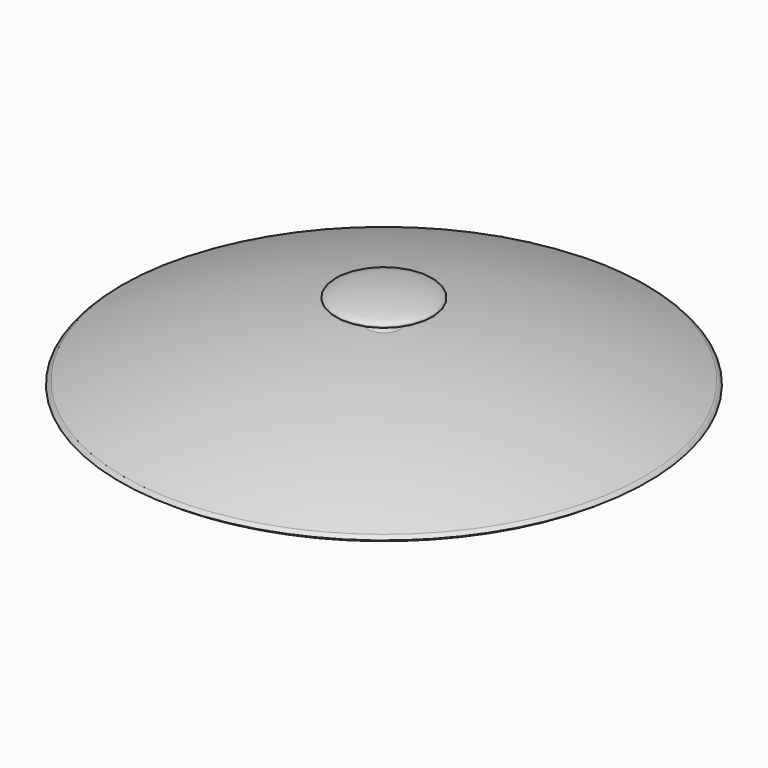
from build123d import *

# Parameters (mm, degrees)
F3_R = 3.175


# Not quite as in the source:
# - a fillet or chamfer that OpenCascade refuses, or shapes differently, is made with other operations: its cross-section is extruded or revolved along the edge and cut away or added


with BuildPart() as f1:
    # F0 (on Front) → F1 (revolve)
    with BuildSketch(Plane.XZ):
        with BuildLine():
            ThreePointArc((-99.06, 0), (-50.3848076923, 13.97), (0, 19.05))
            Line((0, 19.05), (0, 20.9474936326))
            ThreePointArc((0, 20.9474936326), (-1.587572816, 20.9257561642), (-3.175, 20.8951800399))
            ThreePointArc((-3.175, 20.8951800399), (-53.7682024502, 15.2345142884), (-102.54869, 0.6681384411))
            Line((-102.54869, 0.6681384411), (-102.54869, 0))
            Line((-102.54869, 0), (-101.6, 0))
            Line((-101.6, 0), (-99.06, 0))
        make_face()
        with BuildLine():
            ThreePointArc((-101.6, 0), (-100.33, -1.27), (-99.06, 0))
            Line((-99.06, 0), (-101.6, 0))
        make_face()
        with BuildLine():
            ThreePointArc((-3.175, 20.8951800399), (-1.587572816, 20.9257561642), (0, 20.9474936326))
            Line((0, 20.9474936326), (0, 22.8475388139))
            Line((0, 22.8475388139), (0, 27.314457573))
            Line((0, 27.314457573), (-3.175, 27.314457573))
            Line((-3.175, 27.314457573), (-3.175, 20.8951800399))
        make_face()
        with BuildLine():
            Line((-12.7, 27.314457573), (-3.175, 27.314457573))
            Line((-3.175, 27.314457573), (0, 27.314457573))
            Line((0, 27.314457573), (0, 32.8559628492))
            add(Edge.make_bspline(
                [(0, 32.8559628492), (-49.8735474857, 32.8559628492), (-12.7, 27.314457573)],
                knots=[4.7123889804, 4.7123889804, 4.7123889804, 7.1242539777, 7.1242539777, 7.1242539777], degree=2, weights=[1, 0.3568220898, 1]))
        make_face()
    revolve(axis=Axis((0, 0, 16.9409634545), (0, 0, 1)))

    # F2: fillet of radius 3.175 on 1 edges, made by hand

    # F2_s1 → F2_t2 (revolve, cut)
    with BuildSketch(Plane.XZ):
        with BuildLine():
            ThreePointArc((-102.54869, 0), (-101.8842574822, 0.7611764538), (-101.0143260749, 1.2750631254))
            ThreePointArc((-101.0143260749, 1.2750631254), (-101.7819470091, 0.9727105458), (-102.54869, 0.6681384411))
            Line((-102.54869, 0.6681384411), (-102.54869, 0))
        make_face()
    revolve(axis=Axis((0, 0, 0.6681384411), (0, 0, 1)), mode=Mode.SUBTRACT)

    # F3
    f3_edges = [f1.edges().sort_by_distance(p)[0] for p in [
        (3.175, 0, 20.89518),
        (3.175, 0, 27.314458),
    ]]
    fillet(f3_edges, radius=F3_R)


solid = f1.part
